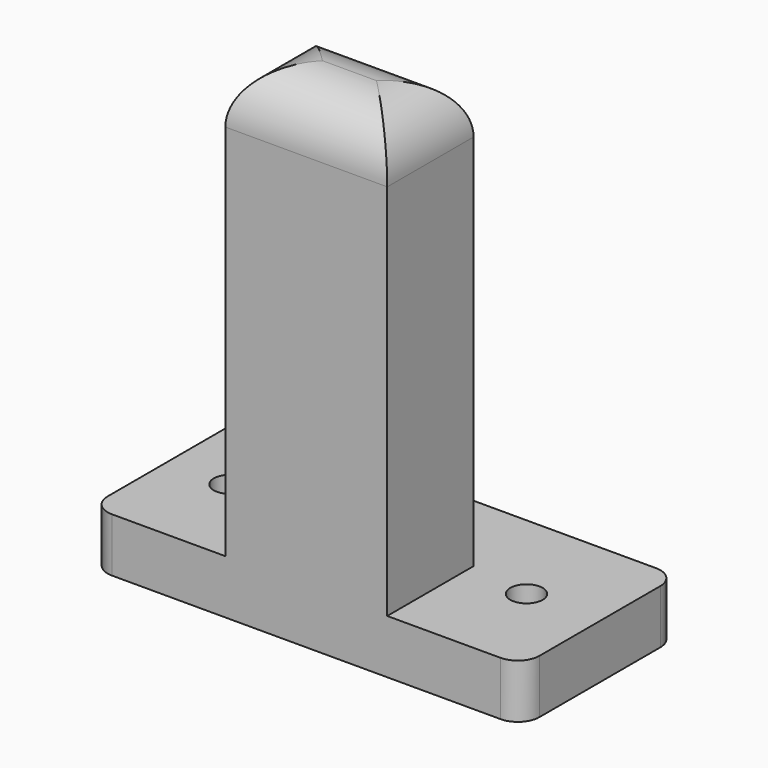
from build123d import *

# Parameters (mm, degrees)
F0_W     = 40
F0_H     = 18
F1_DEPTH = 5
F2_W     = 15
F2_H     = 10
F3_DEPTH = 40
F4_R     = 4.99999
F5_D     = 3
F5_DEPTH = 50
F5_TIP   = 0.9012909285
F6_R     = 2


# Not quite as in the source:
# - a fillet or chamfer is up to 0.001 mm smaller than in the source, because OpenCascade refuses the exact size


with BuildPart() as f1:
    # F0 (on Top) → F1 (new body)
    with BuildSketch(Plane.XY):
        with Locations((-0.0778210488, 9)):
            Rectangle(F0_W, F0_H)
    extrude(amount=F1_DEPTH)

    # F2 (on face) → F3 (join)
    with BuildSketch(Plane.XY.offset(5)):
        with Locations((-0.0778210488, 5)):
            Rectangle(F2_W, F2_H)
    extrude(amount=F3_DEPTH)

    # F4 (radius 5 in the source; OpenCascade refuses exactly that, so slightly less here)
    f4_edges = [f1.edges().sort_by_distance(p)[0] for p in [
        (7.422179, 5, 45),
        (-0.077821, 10, 45),
        (-7.577821, 5, 45),
        (-0.077821, 0, 45),
    ]]
    fillet(f4_edges, radius=F4_R)

    # F5
    with Locations(Plane.XY.offset(5)):
        with Locations((-14.3456859514, 9), (13.1249977276, 9)):
            Hole(F5_D / 2, depth=F5_DEPTH)
            with Locations((0, 0, -(F5_DEPTH + F5_TIP / 2))):  # 118° drill point
                Cone(0, F5_D / 2, F5_TIP, mode=Mode.SUBTRACT)

    # F6
    f6_edges = [f1.edges().sort_by_distance(p)[0] for p in [
        (-20.077821, 0, 2.5),
        (-20.077821, 18, 2.5),
        (19.922179, 18, 2.5),
        (19.922179, 0, 2.5),
    ]]
    fillet(f6_edges, radius=F6_R)


solid = f1.part
